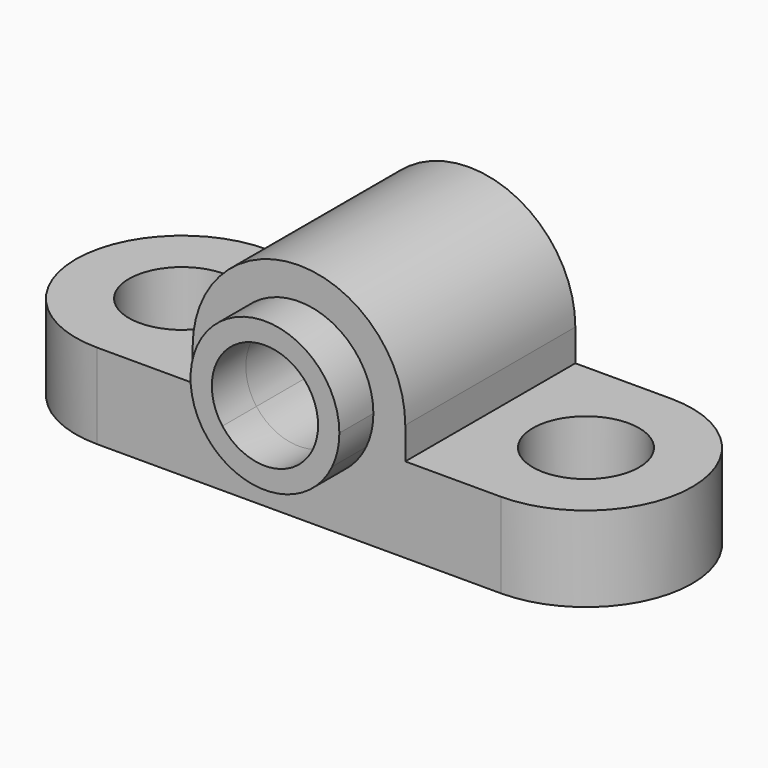
from build123d import *
from build123d import SkipClean  # not in build123d's __all__

# Parameters (mm, degrees)
F0_R     = 5
F1_DEPTH = 8
F3_DEPTH = 20
F4_DEPTH = 20.001
F5_DEPTH = 4


with BuildPart() as f1:
    # F0 (on Top) → F1 (new body)
    with BuildSketch(Plane.XY):
        with BuildLine():
            Line((-19, -10), (19, -10))
            ThreePointArc((19, -10), (29, 0), (19, 10))
            Line((19, 10), (-19, 10))
            ThreePointArc((-19, 10), (-29, 0), (-19, -10))
        make_face()
        with Locations((-19, 0)):
            Circle(F0_R, mode=Mode.SUBTRACT)
        with Locations((19, 0)):
            Circle(F0_R, mode=Mode.SUBTRACT)
    extrude(amount=F1_DEPTH)

    # F2 (on face) → F3 (join, through all)
    with BuildSketch(Plane.XZ.offset(10)):
        with BuildLine():
            Line((-10, 11), (-10, 8))
            Line((-10, 8), (-6.3245553203, 8))
            ThreePointArc((-6.3245553203, 8), (-1.5375488216, 17.8290514437), (7, 11))
            ThreePointArc((7, 11), (6.8290514437, 9.4624511784), (6.3245553203, 8))
            Line((6.3245553203, 8), (10, 8))
            Line((10, 8), (10, 11))
            ThreePointArc((10, 11), (0, 21), (-10, 11))
        make_face()
        with BuildLine():
            Line((-4, 8), (-6.3245553203, 8))
            ThreePointArc((-6.3245553203, 8), (0, 4), (6.3245553203, 8))
            Line((6.3245553203, 8), (4, 8))
            ThreePointArc((4, 8), (0, 6), (-4, 8))
        make_face()
        with BuildLine():
            ThreePointArc((7, 11), (-1.5375488216, 17.8290514437), (-6.3245553203, 8))
            Line((-6.3245553203, 8), (-4, 8))
            ThreePointArc((-4, 8), (-1.5811388301, 15.7434164903), (5, 11))
            ThreePointArc((5, 11), (4.7434164903, 9.4188611699), (4, 8))
            Line((4, 8), (6.3245553203, 8))
            ThreePointArc((6.3245553203, 8), (6.8290514437, 9.4624511784), (7, 11))
        make_face()
    extrude(amount=-F3_DEPTH)

    # F2 (on face) → F4 (cut, through all)
    with BuildSketch(Plane.XZ.offset(10)):
        with BuildLine():
            Line((4, 8), (-4, 8))
            ThreePointArc((-4, 8), (0, 6), (4, 8))
        make_face()
    with SkipClean():  # cleaning this boolean's faces spoils the solid; the shape is the same uncleaned
        extrude(amount=-F4_DEPTH, mode=Mode.SUBTRACT)

    # F2 (on face) → F5 (join)
    with BuildSketch(Plane.XZ.offset(10)):
        with BuildLine():
            Line((-4, 8), (-6.3245553203, 8))
            ThreePointArc((-6.3245553203, 8), (0, 4), (6.3245553203, 8))
            Line((6.3245553203, 8), (4, 8))
            ThreePointArc((4, 8), (0, 6), (-4, 8))
        make_face()
        with BuildLine():
            ThreePointArc((7, 11), (-1.5375488216, 17.8290514437), (-6.3245553203, 8))
            Line((-6.3245553203, 8), (-4, 8))
            ThreePointArc((-4, 8), (-1.5811388301, 15.7434164903), (5, 11))
            ThreePointArc((5, 11), (4.7434164903, 9.4188611699), (4, 8))
            Line((4, 8), (6.3245553203, 8))
            ThreePointArc((6.3245553203, 8), (6.8290514437, 9.4624511784), (7, 11))
        make_face()
    extrude(amount=F5_DEPTH)


solid = f1.part
